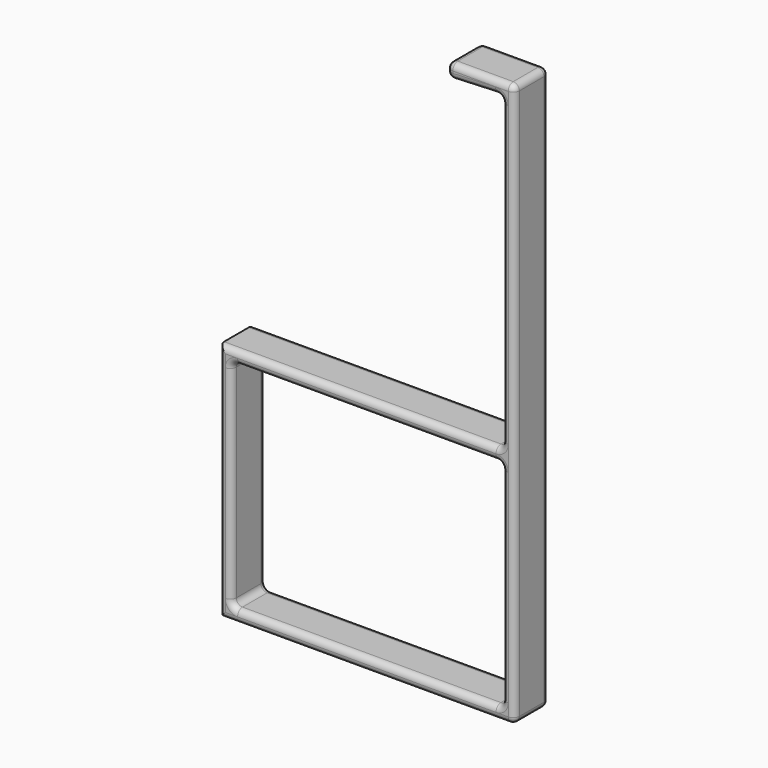
from build123d import *

# Parameters (mm, degrees)
F0_W     = 44
F0_H     = 35
F1_DEPTH = 7
F2_R     = 0.99999


# Not quite as in the source:
# - a fillet or chamfer is up to 0.001 mm smaller than in the source, because OpenCascade refuses the exact size


with BuildPart() as f1:
    # F0 (on Front) → F1 (new body)
    with BuildSketch(Plane.XZ):
        Polygon((-54.2730142517, 66.1785921497), (-54.2730142517, 63.7968573394), (-45.2730142517, 64.1785921497), (-45.2730142517, 13.6785921497), (-91.2730142517, 13.6785921497), (-91.2730142517, 11.6785921497), (-91.2730142517, -23.3214078503), (-91.2730142517, -25.3214078503), (-43.2730142517, -25.3214078503), (-43.2730142517, 66.1785921497), align=None)
        with Locations((-67.2730142517, -5.8214078503)):
            Rectangle(F0_W, F0_H, mode=Mode.SUBTRACT)
    extrude(amount=F1_DEPTH)

    # F2 (radius 1 in the source; OpenCascade refuses exactly that, so slightly less here)
    f2_edges = [f1.edges().sort_by_distance(p)[0] for p in [
        (-48.773014, -7, 66.178592),
        (-54.273014, -7, 64.987725),
        (-49.773014, -7, 63.987725),
        (-45.273014, -7, 38.928592),
        (-68.273014, -7, 13.678592),
        (-91.273014, -7, -5.821408),
        (-67.273014, -7, -25.321408),
        (-43.273014, -7, 20.428592),
        (-45.273014, -7, -5.821408),
        (-67.273014, -7, -23.321408),
        (-89.273014, -7, -5.821408),
        (-67.273014, -7, 11.678592),
        (-48.773014, 0, 66.178592),
        (-54.273014, 0, 64.987725),
        (-49.773014, 0, 63.987725),
        (-45.273014, 0, 38.928592),
        (-68.273014, 0, 13.678592),
        (-91.273014, 0, -5.821408),
        (-67.273014, 0, -25.321408),
        (-43.273014, 0, 20.428592),
        (-45.273014, 0, -5.821408),
        (-67.273014, 0, -23.321408),
        (-89.273014, 0, -5.821408),
        (-67.273014, 0, 11.678592),
        (-45.273014, -3.5, 11.678592),
        (-45.273014, -3.5, -23.321408),
        (-89.273014, -3.5, 11.678592),
        (-89.273014, -3.5, -23.321408),
        (-54.273014, -3.5, 63.796857),
        (-45.273014, -3.5, 64.178592),
        (-54.273014, -3.5, 66.178592),
        (-43.273014, -3.5, 66.178592),
        (-45.273014, -3.5, 13.678592),
        (-43.273014, -3.5, -25.321408),
    ]]
    fillet(f2_edges, radius=F2_R)


solid = f1.part
